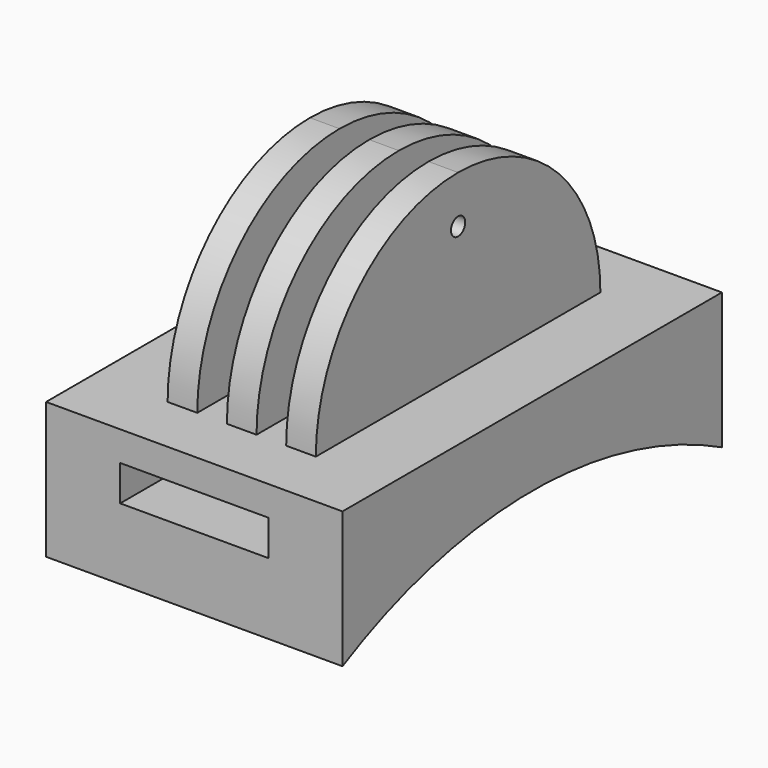
from build123d import *

# Parameters (mm, degrees)
F0_W      = 50
F0_H      = 80
F1_DEPTH  = 6
F2_W      = 5
F2_H      = 60
F3_DEPTH  = 30
F4_R      = 29.99999
F5_DEPTH  = 40
F7_DEPTH  = 65
F8_W      = 25
F8_H      = 6
F9_DEPTH  = 115.9
F10_R     = 1.5
F11_DEPTH = 30.7


# Not quite as in the source:
# - a fillet or chamfer is up to 0.001 mm smaller than in the source, because OpenCascade refuses the exact size


with BuildPart() as f1:
    # F0 (on Top) → F1 (new body)
    with BuildSketch(Plane.XY):
        Rectangle(F0_W, F0_H)
    extrude(amount=F1_DEPTH)

    # F2 (on face) → F3 (join)
    with BuildSketch(Plane.XY.offset(6)):
        Rectangle(F2_W, F2_H)
        with Locations((-10, 0)):
            Rectangle(F2_W, F2_H)
        with Locations((10, 0)):
            Rectangle(F2_W, F2_H)
    extrude(amount=F3_DEPTH)

    # F4 (radius 30 in the source; OpenCascade refuses exactly that, so slightly less here)
    f4_edges = [f1.edges().sort_by_distance(p)[0] for p in [
        (10, 30, 36),
        (0, 30, 36),
        (-10, 30, 36),
        (-10, -30, 36),
        (0, -30, 36),
        (10, -30, 36),
    ]]
    fillet(f4_edges, radius=F4_R)

    # F5 (add): a face of the model
    f5_faces = [f1.faces().sort_by_distance(p)[0] for p in [
        (0, 0, 0),
    ]]
    extrude(f5_faces, amount=F5_DEPTH)

    # F6 (on face) → F7 (cut)
    with BuildSketch(Plane(origin=(-25, 0, 0), x_dir=(0, -1, 0), z_dir=(-1, 0, 0))):
        with BuildLine():
            Line((40, -40), (40, -17))
            ThreePointArc((40, -17), (0, -7.2132285382), (-40, -17))
            Line((-40, -17), (-40, -40))
            Line((-40, -40), (40, -40))
        make_face()
    extrude(amount=-F7_DEPTH, mode=Mode.SUBTRACT)

    # F8 (on face) → F9 (cut)
    with BuildSketch(Plane(origin=(0, 40, 0), x_dir=(-1, 0, 0), z_dir=(0, 1, 0))):
        with Locations((0, -2)):
            Rectangle(F8_W, F8_H)
    extrude(amount=-F9_DEPTH, mode=Mode.SUBTRACT)

    # F10 (on face) → F11 (cut)
    with BuildSketch(Plane(origin=(-12.5, 0, 0), x_dir=(0, -1, 0), z_dir=(-1, 0, 0))):
        with Locations((0, 28)):
            Circle(F10_R)
    extrude(amount=-F11_DEPTH, mode=Mode.SUBTRACT)


solid = f1.part
